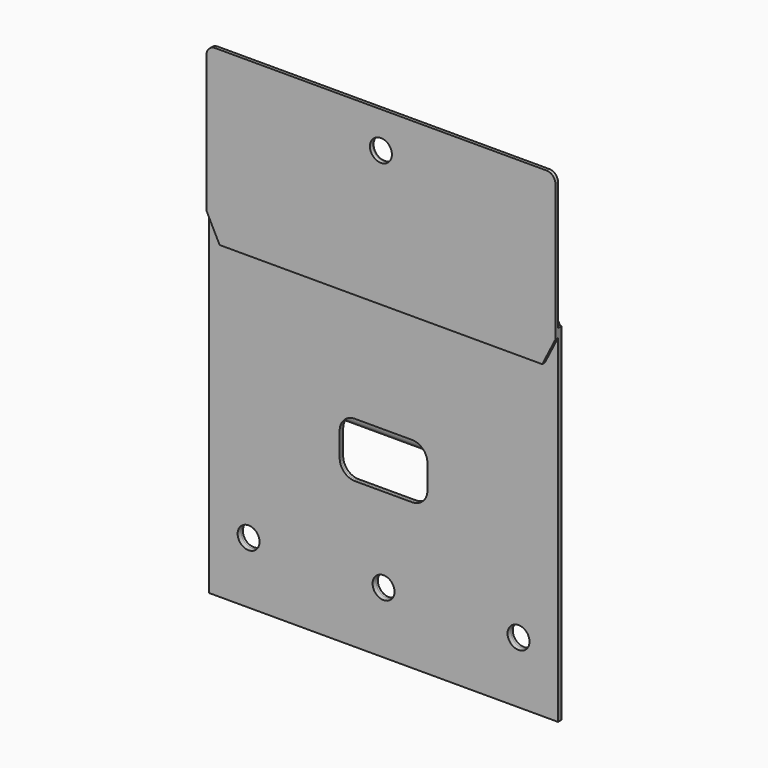
from build123d import *

# Parameters (mm, degrees)
F1_DEPTH = 5
F2_R     = 4.5
F3_R     = 5
F4_DEPTH = 2
F5_DEPTH = 1
F6_R     = 5
F7_DEPTH = 1.5
F8_DEPTH = 0.55
F9_DEPTH = 1


# Not quite as in the source:
# - a feature names something its author has since deleted; it is built from what else it names


with BuildPart() as f1:
    # F0 (on Front) → F1 (new body, symmetric)
    with BuildSketch(Plane.XZ):
        with BuildLine():
            ThreePointArc((73.5, 28), (71.1568542495, 33.6568542495), (65.5, 36))
            Line((65.5, 36), (-65.5, 36))
            ThreePointArc((-65.5, 36), (-71.1568542495, 33.6568542495), (-73.5, 28))
            Line((-73.5, 28), (-73.5, -28))
            ThreePointArc((-73.5, -28), (-71.1568542495, -33.6568542495), (-65.5, -36))
            Line((-65.5, -36), (65.5, -36))
            ThreePointArc((65.5, -36), (71.1568542495, -33.6568542495), (73.5, -28))
            Line((73.5, -28), (73.5, 28))
        make_face()
    extrude(amount=F1_DEPTH, both=True)

    # F2
    f2_edges = [f1.edges().sort_by_distance(p)[0] for p in [
        (71.156854, -5, 33.656854),
        (0, -5, 36),
        (-71.156854, -5, 33.656854),
        (-73.5, -5, 0),
        (-71.156854, -5, -33.656854),
        (0, -5, -36),
        (71.156854, -5, -33.656854),
        (73.5, -5, 0),
        (71.156854, 5, 33.656854),
        (0, 5, 36),
        (-71.156854, 5, 33.656854),
        (-73.5, 5, 0),
        (-71.156854, 5, -33.656854),
        (0, 5, -36),
        (71.156854, 5, -33.656854),
        (73.5, 5, 0),
    ]]
    fillet(f2_edges, radius=F2_R)


with BuildPart() as f4:
    # F3 (on face) → F4 (new body)
    with BuildSketch(Plane.XZ.offset(5)):
        Polygon((65.5, 36), (-65.5, 36), (-79.5, 36), (-79.5, -122), (79.5, -122), (79.5, 36), align=None)
        with BuildLine():
            Line((-73.5, -50), (-24.9058808998, -50))
            ThreePointArc((-24.9058808998, -50), (-20.9372539332, -57.5), (-13, -60.5))
            Line((-13, -60.5), (13, -60.5))
            ThreePointArc((13, -60.5), (20.9372539332, -57.5), (24.9058808998, -50))
            Line((24.9058808998, -50), (73.5, -50))
            Line((73.5, -50), (73.5, -118))
            Line((73.5, -118), (-73.5, -118))
            Line((-73.5, -118), (-73.5, -50))
        make_face(mode=Mode.SUBTRACT)
        with BuildLine():
            ThreePointArc((-20, -37.5), (-17.9497474683, -32.5502525317), (-13, -30.5))
            Line((-13, -30.5), (13, -30.5))
            ThreePointArc((13, -30.5), (17.9497474683, -32.5502525317), (20, -37.5))
            Line((20, -37.5), (20, -48.5))
            ThreePointArc((20, -48.5), (17.9497474683, -53.4497474683), (13, -55.5))
            Line((13, -55.5), (-13, -55.5))
            ThreePointArc((-13, -55.5), (-17.9497474683, -53.4497474683), (-20, -48.5))
            Line((-20, -48.5), (-20, -37.5))
        make_face(mode=Mode.SUBTRACT)
        with BuildLine():
            Line((73.5, 32), (73.5, -36))
            Line((73.5, -36), (24.9058808998, -36))
            ThreePointArc((24.9058808998, -36), (20.9372539332, -28.5), (13, -25.5))
            Line((13, -25.5), (-13, -25.5))
            ThreePointArc((-13, -25.5), (-20.9372539332, -28.5), (-24.9058808998, -36))
            Line((-24.9058808998, -36), (-73.5, -36))
            Line((-73.5, -36), (-73.5, 32))
            Line((-73.5, 32), (73.5, 32))
        make_face(mode=Mode.SUBTRACT)
        with BuildLine():
            ThreePointArc((13, -25.5), (19, -27.1076951546), (23.3923048454, -31.5))
            Line((23.3923048454, -31.5), (65.5, -31.5))
            ThreePointArc((65.5, -31.5), (67.9748737342, -30.4748737342), (69, -28))
            Line((69, -28), (69, 28))
            ThreePointArc((69, 28), (67.9748737342, 30.4748737342), (65.5, 31.5))
            Line((65.5, 31.5), (-65.5, 31.5))
            ThreePointArc((-65.5, 31.5), (-67.9748737342, 30.4748737342), (-69, 28))
            Line((-69, 28), (-69, -28))
            ThreePointArc((-69, -28), (-67.9748737342, -30.4748737342), (-65.5, -31.5))
            Line((-65.5, -31.5), (-23.3923048454, -31.5))
            ThreePointArc((-23.3923048454, -31.5), (-19, -27.1076951546), (-13, -25.5))
            Line((-13, -25.5), (13, -25.5))
        make_face()
        with BuildLine():
            ThreePointArc((-13, -60.5), (-20.9372539332, -57.5), (-24.9058808998, -50))
            Line((-24.9058808998, -50), (-73.5, -50))
            Line((-73.5, -50), (-73.5, -118))
            Line((-73.5, -118), (73.5, -118))
            Line((73.5, -118), (73.5, -50))
            Line((73.5, -50), (24.9058808998, -50))
            ThreePointArc((24.9058808998, -50), (20.9372539332, -57.5), (13, -60.5))
            Line((13, -60.5), (-13, -60.5))
        make_face()
        with Locations((-61.5, -94)):
            Circle(F3_R, mode=Mode.SUBTRACT)
        with Locations((0, -94)):
            Circle(F3_R, mode=Mode.SUBTRACT)
        with Locations((61.5, -94)):
            Circle(F3_R, mode=Mode.SUBTRACT)
        with BuildLine():
            Line((24.9058808998, -36), (73.5, -36))
            Line((73.5, -36), (73.5, 32))
            Line((73.5, 32), (-73.5, 32))
            Line((-73.5, 32), (-73.5, -36))
            Line((-73.5, -36), (-24.9058808998, -36))
            ThreePointArc((-24.9058808998, -36), (-24.3738635424, -33.6743983325), (-23.3923048454, -31.5))
            Line((-23.3923048454, -31.5), (-65.5, -31.5))
            ThreePointArc((-65.5, -31.5), (-67.9748737342, -30.4748737342), (-69, -28))
            Line((-69, -28), (-69, 28))
            ThreePointArc((-69, 28), (-67.9748737342, 30.4748737342), (-65.5, 31.5))
            Line((-65.5, 31.5), (65.5, 31.5))
            ThreePointArc((65.5, 31.5), (67.9748737342, 30.4748737342), (69, 28))
            Line((69, 28), (69, -28))
            ThreePointArc((69, -28), (67.9748737342, -30.4748737342), (65.5, -31.5))
            Line((65.5, -31.5), (23.3923048454, -31.5))
            ThreePointArc((23.3923048454, -31.5), (24.3738635424, -33.6743983325), (24.9058808998, -36))
        make_face()
    extrude(amount=F4_DEPTH)


with BuildPart() as f5:
    # F3 (on face) → F5 (new body)
    with BuildSketch(Plane.XZ.offset(5)):
        with BuildLine():
            Line((24.9058808998, -36), (73.5, -36))
            Line((73.5, -36), (73.5, 32))
            Line((73.5, 32), (-73.5, 32))
            Line((-73.5, 32), (-73.5, -36))
            Line((-73.5, -36), (-24.9058808998, -36))
            ThreePointArc((-24.9058808998, -36), (-24.3738635424, -33.6743983325), (-23.3923048454, -31.5))
            Line((-23.3923048454, -31.5), (-65.5, -31.5))
            ThreePointArc((-65.5, -31.5), (-67.9748737342, -30.4748737342), (-69, -28))
            Line((-69, -28), (-69, 28))
            ThreePointArc((-69, 28), (-67.9748737342, 30.4748737342), (-65.5, 31.5))
            Line((-65.5, 31.5), (65.5, 31.5))
            ThreePointArc((65.5, 31.5), (67.9748737342, 30.4748737342), (69, 28))
            Line((69, 28), (69, -28))
            ThreePointArc((69, -28), (67.9748737342, -30.4748737342), (65.5, -31.5))
            Line((65.5, -31.5), (23.3923048454, -31.5))
            ThreePointArc((23.3923048454, -31.5), (24.3738635424, -33.6743983325), (24.9058808998, -36))
        make_face()
        with BuildLine():
            ThreePointArc((13, -25.5), (19, -27.1076951546), (23.3923048454, -31.5))
            Line((23.3923048454, -31.5), (65.5, -31.5))
            ThreePointArc((65.5, -31.5), (67.9748737342, -30.4748737342), (69, -28))
            Line((69, -28), (69, 28))
            ThreePointArc((69, 28), (67.9748737342, 30.4748737342), (65.5, 31.5))
            Line((65.5, 31.5), (-65.5, 31.5))
            ThreePointArc((-65.5, 31.5), (-67.9748737342, 30.4748737342), (-69, 28))
            Line((-69, 28), (-69, -28))
            ThreePointArc((-69, -28), (-67.9748737342, -30.4748737342), (-65.5, -31.5))
            Line((-65.5, -31.5), (-23.3923048454, -31.5))
            ThreePointArc((-23.3923048454, -31.5), (-19, -27.1076951546), (-13, -25.5))
            Line((-13, -25.5), (13, -25.5))
        make_face()
    extrude(amount=-F5_DEPTH)


with BuildPart() as f5b:
    # F3 (on face) → F5, piece 2 (new body)
    with BuildSketch(Plane.XZ.offset(5)):
        with BuildLine():
            ThreePointArc((-13, -60.5), (-20.9372539332, -57.5), (-24.9058808998, -50))
            Line((-24.9058808998, -50), (-73.5, -50))
            Line((-73.5, -50), (-73.5, -118))
            Line((-73.5, -118), (73.5, -118))
            Line((73.5, -118), (73.5, -50))
            Line((73.5, -50), (24.9058808998, -50))
            ThreePointArc((24.9058808998, -50), (20.9372539332, -57.5), (13, -60.5))
            Line((13, -60.5), (-13, -60.5))
        make_face()
        with Locations((-61.5, -94)):
            Circle(F3_R, mode=Mode.SUBTRACT)
        with Locations((0, -94)):
            Circle(F3_R, mode=Mode.SUBTRACT)
        with Locations((61.5, -94)):
            Circle(F3_R, mode=Mode.SUBTRACT)
    extrude(amount=-F5_DEPTH)


with BuildPart() as f7:
    # F6 (on face) → F7 (new body)
    with BuildSketch(Plane.XZ.offset(7)):
        with BuildLine():
            ThreePointArc((-75.5, 98.496), (-78.3284271247, 97.3244271247), (-79.5, 94.496))
            Line((-79.5, 94.496), (-79.5, 36))
            Line((-79.5, 36), (79.5, 36))
            Line((79.5, 36), (79.5, 94.496))
            ThreePointArc((79.5, 94.496), (78.3284271247, 97.3244271247), (75.5, 98.496))
            Line((75.5, 98.496), (0, 98.496))
            Line((0, 98.496), (-75.5, 98.496))
        make_face()
        with BuildLine():
            Line((73.5, 54), (-73.5, 54))
            Line((-73.5, 54), (-73.5, 92.996))
            ThreePointArc((-73.5, 92.996), (-73.0606601718, 94.0566601718), (-72, 94.496))
            Line((-72, 94.496), (72, 94.496))
            ThreePointArc((72, 94.496), (73.0606601718, 94.0566601718), (73.5, 92.996))
            Line((73.5, 92.996), (73.5, 54))
        make_face(mode=Mode.SUBTRACT)
        Polygon((79.5, 36), (-79.5, 36), (-79.5, 32), (-73.5, 20.16), (0, 20.16), (73.5, 20.16), (79.5, 32), align=None)
        with BuildLine():
            Line((-73.5, 92.996), (-73.5, 54))
            Line((-73.5, 54), (73.5, 54))
            Line((73.5, 54), (73.5, 92.996))
            ThreePointArc((73.5, 92.996), (73.0606601718, 94.0566601718), (72, 94.496))
            Line((72, 94.496), (-72, 94.496))
            ThreePointArc((-72, 94.496), (-73.0606601718, 94.0566601718), (-73.5, 92.996))
        make_face()
        with Locations((-61.5, 82)):
            Circle(F6_R, mode=Mode.SUBTRACT)
        with Locations((0, 82)):
            Circle(F6_R, mode=Mode.SUBTRACT)
        with Locations((61.5, 82)):
            Circle(F6_R, mode=Mode.SUBTRACT)
        with Locations((61.5, 82)):
            Circle(F6_R)
        with Locations((-61.5, 82)):
            Circle(F6_R)
    extrude(amount=F7_DEPTH)


with BuildPart() as f8:
    # F6 (on face) → F8 (new body)
    with BuildSketch(Plane.XZ.offset(7)):
        with BuildLine():
            Line((-73.5, 92.996), (-73.5, 54))
            Line((-73.5, 54), (73.5, 54))
            Line((73.5, 54), (73.5, 92.996))
            ThreePointArc((73.5, 92.996), (73.0606601718, 94.0566601718), (72, 94.496))
            Line((72, 94.496), (-72, 94.496))
            ThreePointArc((-72, 94.496), (-73.0606601718, 94.0566601718), (-73.5, 92.996))
        make_face()
        with Locations((-61.5, 82)):
            Circle(F6_R, mode=Mode.SUBTRACT)
        with Locations((0, 82)):
            Circle(F6_R, mode=Mode.SUBTRACT)
        with Locations((61.5, 82)):
            Circle(F6_R, mode=Mode.SUBTRACT)
    extrude(amount=-F8_DEPTH)


with BuildPart() as f9:
    # F3 (on face) → F9 (new body)
    with BuildSketch(Plane.XZ.offset(5)):
        Polygon((65.5, 36), (-65.5, 36), (-79.5, 36), (-79.5, -122), (79.5, -122), (79.5, 36), align=None)
        with BuildLine():
            Line((-73.5, -50), (-24.9058808998, -50))
            ThreePointArc((-24.9058808998, -50), (-20.9372539332, -57.5), (-13, -60.5))
            Line((-13, -60.5), (13, -60.5))
            ThreePointArc((13, -60.5), (20.9372539332, -57.5), (24.9058808998, -50))
            Line((24.9058808998, -50), (73.5, -50))
            Line((73.5, -50), (73.5, -118))
            Line((73.5, -118), (-73.5, -118))
            Line((-73.5, -118), (-73.5, -50))
        make_face(mode=Mode.SUBTRACT)
        with BuildLine():
            ThreePointArc((-20, -37.5), (-17.9497474683, -32.5502525317), (-13, -30.5))
            Line((-13, -30.5), (13, -30.5))
            ThreePointArc((13, -30.5), (17.9497474683, -32.5502525317), (20, -37.5))
            Line((20, -37.5), (20, -48.5))
            ThreePointArc((20, -48.5), (17.9497474683, -53.4497474683), (13, -55.5))
            Line((13, -55.5), (-13, -55.5))
            ThreePointArc((-13, -55.5), (-17.9497474683, -53.4497474683), (-20, -48.5))
            Line((-20, -48.5), (-20, -37.5))
        make_face(mode=Mode.SUBTRACT)
        with BuildLine():
            Line((73.5, 32), (73.5, -36))
            Line((73.5, -36), (24.9058808998, -36))
            ThreePointArc((24.9058808998, -36), (20.9372539332, -28.5), (13, -25.5))
            Line((13, -25.5), (-13, -25.5))
            ThreePointArc((-13, -25.5), (-20.9372539332, -28.5), (-24.9058808998, -36))
            Line((-24.9058808998, -36), (-73.5, -36))
            Line((-73.5, -36), (-73.5, 32))
            Line((-73.5, 32), (73.5, 32))
        make_face(mode=Mode.SUBTRACT)
        with BuildLine():
            Line((24.9058808998, -36), (73.5, -36))
            Line((73.5, -36), (73.5, 32))
            Line((73.5, 32), (-73.5, 32))
            Line((-73.5, 32), (-73.5, -36))
            Line((-73.5, -36), (-24.9058808998, -36))
            ThreePointArc((-24.9058808998, -36), (-24.3738635424, -33.6743983325), (-23.3923048454, -31.5))
            Line((-23.3923048454, -31.5), (-65.5, -31.5))
            ThreePointArc((-65.5, -31.5), (-67.9748737342, -30.4748737342), (-69, -28))
            Line((-69, -28), (-69, 28))
            ThreePointArc((-69, 28), (-67.9748737342, 30.4748737342), (-65.5, 31.5))
            Line((-65.5, 31.5), (65.5, 31.5))
            ThreePointArc((65.5, 31.5), (67.9748737342, 30.4748737342), (69, 28))
            Line((69, 28), (69, -28))
            ThreePointArc((69, -28), (67.9748737342, -30.4748737342), (65.5, -31.5))
            Line((65.5, -31.5), (23.3923048454, -31.5))
            ThreePointArc((23.3923048454, -31.5), (24.3738635424, -33.6743983325), (24.9058808998, -36))
        make_face()
        with BuildLine():
            ThreePointArc((13, -25.5), (19, -27.1076951546), (23.3923048454, -31.5))
            Line((23.3923048454, -31.5), (65.5, -31.5))
            ThreePointArc((65.5, -31.5), (67.9748737342, -30.4748737342), (69, -28))
            Line((69, -28), (69, 28))
            ThreePointArc((69, 28), (67.9748737342, 30.4748737342), (65.5, 31.5))
            Line((65.5, 31.5), (-65.5, 31.5))
            ThreePointArc((-65.5, 31.5), (-67.9748737342, 30.4748737342), (-69, 28))
            Line((-69, 28), (-69, -28))
            ThreePointArc((-69, -28), (-67.9748737342, -30.4748737342), (-65.5, -31.5))
            Line((-65.5, -31.5), (-23.3923048454, -31.5))
            ThreePointArc((-23.3923048454, -31.5), (-19, -27.1076951546), (-13, -25.5))
            Line((-13, -25.5), (13, -25.5))
        make_face()
    extrude(amount=F9_DEPTH)


solid = Compound([f1.part, f4.part, f5.part, f5b.part, f7.part, f8.part, f9.part])
